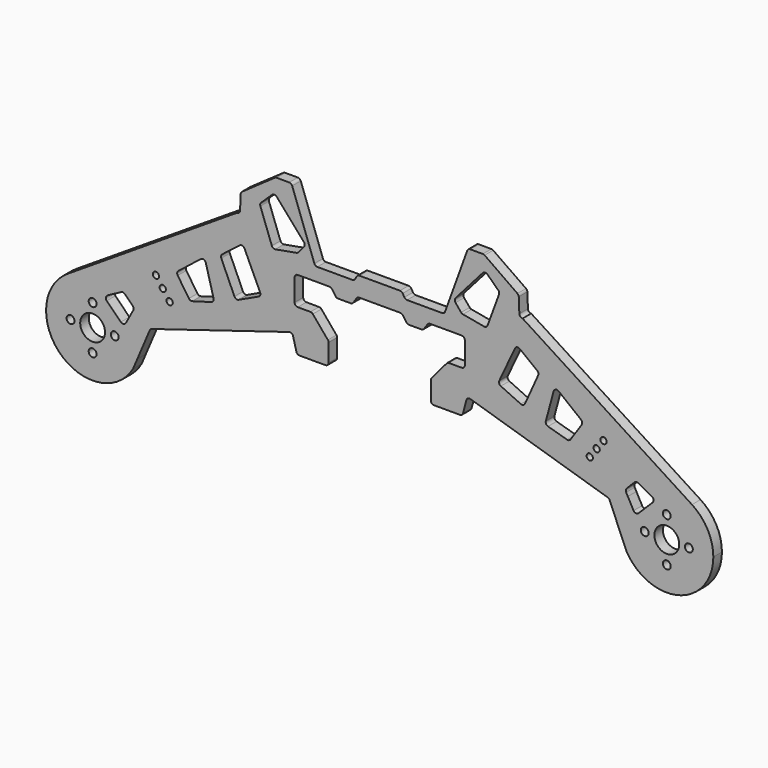
from build123d import *

# Parameters (mm, degrees)
F0_R     = 1
F0_R_2   = 1.25
F0_R_3   = 3.9333333333
F1_DEPTH = 3.4


# Not quite as in the source:
# - a feature names something its author has since deleted; it is built from what else it names


with BuildPart() as f1:
    # F0 (on Front) → F1 (new body)
    with BuildSketch(Plane.XZ):
        with BuildLine():
            Line((-8.2982365832, 14.9417242708), (-61.9791285384, 49.42693132))
            ThreePointArc((-61.9791285384, 49.42693132), (-62.6848131058, 49.6987576936), (-62.9984126547, 50.3868969303))
            Line((-62.9984126547, 50.3868969303), (-63.1852708125, 55.0742351752))
            ThreePointArc((-63.1852708125, 55.0742351752), (-63.3068405454, 55.5137289261), (-63.6109007347, 55.8535544083))
            Line((-63.6109007347, 55.8535544083), (-74.0052830565, 63.131779265))
            ThreePointArc((-74.0052830565, 63.131779265), (-74.2781536934, 63.2663441715), (-74.5788594929, 63.3126272207))
            Line((-74.5788594929, 63.3126272207), (-78.5633531658, 63.3126272207))
            ThreePointArc((-78.5633531658, 63.3126272207), (-79.1369296021, 63.131779265), (-79.5030457866, 62.6546473641))
            Line((-79.5030457866, 62.6546473641), (-86.5485187746, 43.2973694201))
            ThreePointArc((-86.5485187746, 43.2973694201), (-86.914634959, 42.8202375192), (-87.4882113954, 42.6393895635))
            Line((-87.4882113954, 42.6393895635), (-98.5779405442, 42.6393895635))
            ThreePointArc((-98.5779405442, 42.6393895635), (-99.0779405442, 42.7733641597), (-99.443965948, 43.1393895635))
            Line((-99.443965948, 43.1393895635), (-99.9635811902, 44.0393895635))
            ThreePointArc((-99.9635811902, 44.0393895635), (-100.329606594, 44.4054149672), (-100.829606594, 44.5393895635))
            Line((-100.829606594, 44.5393895635), (-107.2522563248, 44.5393895635))
            Line((-107.2522563248, 44.5393895635), (-113.6749060556, 44.5393895635))
            ThreePointArc((-113.6749060556, 44.5393895635), (-114.1749060556, 44.4054149672), (-114.5409314594, 44.0393895635))
            Line((-114.5409314594, 44.0393895635), (-115.0605467017, 43.1393895635))
            ThreePointArc((-115.0605467017, 43.1393895635), (-115.4265721055, 42.7733641597), (-115.9265721055, 42.6393895635))
            Line((-115.9265721055, 42.6393895635), (-127.0163012543, 42.6393895635))
            ThreePointArc((-127.0163012543, 42.6393895635), (-127.5898776906, 42.8202375192), (-127.9559938751, 43.2973694201))
            Line((-127.9559938751, 43.2973694201), (-135.0014668631, 62.6546473641))
            ThreePointArc((-135.0014668631, 62.6546473641), (-135.3675830475, 63.131779265), (-135.9411594839, 63.3126272207))
            Line((-135.9411594839, 63.3126272207), (-139.9256531568, 63.3126272207))
            ThreePointArc((-139.9256531568, 63.3126272207), (-140.2263589563, 63.2663441715), (-140.4992295931, 63.131779265))
            Line((-140.4992295931, 63.131779265), (-150.8936119149, 55.8535544083))
            ThreePointArc((-150.8936119149, 55.8535544083), (-151.1976721043, 55.5137289261), (-151.3192418372, 55.0742351752))
            Line((-151.3192418372, 55.0742351752), (-151.5060999949, 50.3868969303))
            ThreePointArc((-151.5060999949, 50.3868969303), (-151.8196995438, 49.6987576936), (-152.5253841113, 49.42693132))
            Line((-152.5253841113, 49.42693132), (-206.2062760664, 14.9417242708))
            ThreePointArc((-206.2062760664, 14.9417242708), (-198.1780596026, 17.281718999), (-190.1678289018, 14.8808776804))
            Line((-190.1678289018, 14.8808776804), (-189.1965146494, 15.4060313881))
            ThreePointArc((-189.1965146494, 15.4060313881), (-188.576544649, 15.5158937889), (-188.01380745, 15.2334767332))
            Line((-188.01380745, 15.2334767332), (-185.5323660974, 12.7520353807))
            ThreePointArc((-185.5323660974, 12.7520353807), (-185.2499490417, 12.1892981816), (-185.3598114425, 11.5693281812))
            Line((-185.3598114425, 11.5693281812), (-185.8849651503, 10.5980139288))
            ThreePointArc((-185.8849651503, 10.5980139288), (-184.0969913909, 6.7397922977), (-183.4840176852, 2.5318251454))
            ThreePointArc((-183.4840176852, 2.5318251454), (-183.6340282552, 0.4335380721), (-184.0810086875, -1.6220689687))
            Line((-184.0810086875, -1.6220689687), (-180.1264152738, 7.694369281))
            ThreePointArc((-180.1264152738, 7.694369281), (-179.8750410267, 8.0467829779), (-179.4982821251, 8.2599429084))
            Line((-179.4982821251, 8.2599429084), (-135.98817339, 21.5623181023))
            ThreePointArc((-135.98817339, 21.5623181023), (-135.2109920651, 21.4806330535), (-134.729875859, 20.8648323915))
            Line((-134.729875859, 20.8648323915), (-133.6435753937, 16.8107038626))
            ThreePointArc((-133.6435753937, 16.8107038626), (-133.2864109964, 16.2761695674), (-132.6776495674, 16.0695229077))
            Line((-132.6776495674, 16.0695229077), (-124.4449765554, 16.0695229077))
            ThreePointArc((-124.4449765554, 16.0695229077), (-123.7378697742, 16.3624161265), (-123.4449765554, 17.0695229077))
            Line((-123.4449765554, 17.0695229077), (-123.4449765554, 22.7055526735))
            ThreePointArc((-123.4449765554, 22.7055526735), (-123.5052839346, 23.0475728168), (-123.6789321123, 23.3483402831))
            Line((-123.6789321123, 23.3483402831), (-128.4482375504, 29.0321771731))
            ThreePointArc((-128.4482375504, 29.0321771731), (-128.7916637317, 29.2956973505), (-129.2142819935, 29.3893895635))
            Line((-129.2142819935, 29.3893895635), (-133.2142819935, 29.3893895635))
            ThreePointArc((-133.2142819935, 29.3893895635), (-133.9213887747, 29.6822827823), (-134.2142819935, 30.3893895635))
            Line((-134.2142819935, 30.3893895635), (-134.2142819935, 37.3893895635))
            ThreePointArc((-134.2142819935, 37.3893895635), (-133.9213887747, 38.0964963446), (-133.2142819935, 38.3893895635))
            Line((-133.2142819935, 38.3893895635), (-123.2142819935, 38.3893895635))
            ThreePointArc((-123.2142819935, 38.3893895635), (-122.7525333802, 38.2764003966), (-122.3951299492, 37.9629659998))
            Line((-122.3951299492, 37.9629659998), (-121.2715706276, 36.3583569942))
            ThreePointArc((-121.2715706276, 36.3583569942), (-120.9141671966, 36.0449225974), (-120.4524185833, 35.9319334306))
            Line((-120.4524185833, 35.9319334306), (-116.4935526844, 35.9319334306))
            ThreePointArc((-116.4935526844, 35.9319334306), (-116.0318040712, 36.0449225974), (-115.6744006401, 36.3583569942))
            Line((-115.6744006401, 36.3583569942), (-114.5508413186, 37.9629659998))
            ThreePointArc((-114.5508413186, 37.9629659998), (-114.1934378875, 38.2764003966), (-113.7316892743, 38.3893895635))
            Line((-113.7316892743, 38.3893895635), (-107.2522563248, 38.3893895635))
            Line((-107.2522563248, 38.3893895635), (-100.7728233754, 38.3893895635))
            ThreePointArc((-100.7728233754, 38.3893895635), (-100.3110747621, 38.2764003966), (-99.9536713311, 37.9629659998))
            Line((-99.9536713311, 37.9629659998), (-98.8301120095, 36.3583569942))
            ThreePointArc((-98.8301120095, 36.3583569942), (-98.4727085785, 36.0449225974), (-98.0109599652, 35.9319334306))
            Line((-98.0109599652, 35.9319334306), (-94.0520940663, 35.9319334306))
            ThreePointArc((-94.0520940663, 35.9319334306), (-93.5903454531, 36.0449225974), (-93.232942022, 36.3583569942))
            Line((-93.232942022, 36.3583569942), (-92.1093827005, 37.9629659998))
            ThreePointArc((-92.1093827005, 37.9629659998), (-91.7519792694, 38.2764003966), (-91.2902306562, 38.3893895635))
            Line((-91.2902306562, 38.3893895635), (-81.2902306562, 38.3893895635))
            ThreePointArc((-81.2902306562, 38.3893895635), (-80.583123875, 38.0964963446), (-80.2902306562, 37.3893895635))
            Line((-80.2902306562, 37.3893895635), (-80.2902306562, 30.3893895635))
            ThreePointArc((-80.2902306562, 30.3893895635), (-80.583123875, 29.6822827823), (-81.2902306562, 29.3893895635))
            Line((-81.2902306562, 29.3893895635), (-85.2902306562, 29.3893895635))
            ThreePointArc((-85.2902306562, 29.3893895635), (-85.7128489179, 29.2956973505), (-86.0562750993, 29.0321771731))
            Line((-86.0562750993, 29.0321771731), (-90.8255805374, 23.3483402831))
            ThreePointArc((-90.8255805374, 23.3483402831), (-90.999228715, 23.0475728168), (-91.0595360942, 22.7055526735))
            Line((-91.0595360942, 22.7055526735), (-91.0595360942, 17.0695229077))
            ThreePointArc((-91.0595360942, 17.0695229077), (-90.7666428754, 16.3624161265), (-90.0595360942, 16.0695229077))
            Line((-90.0595360942, 16.0695229077), (-81.8268630822, 16.0695229077))
            ThreePointArc((-81.8268630822, 16.0695229077), (-81.2181016532, 16.2761695674), (-80.8609372559, 16.8107038626))
            Line((-80.8609372559, 16.8107038626), (-79.7746367906, 20.8648323915))
            ThreePointArc((-79.7746367906, 20.8648323915), (-79.2935205846, 21.4806330535), (-78.5163392596, 21.5623181023))
            Line((-78.5163392596, 21.5623181023), (-35.0062305246, 8.2599429084))
            ThreePointArc((-35.0062305246, 8.2599429084), (-34.629471623, 8.0467829779), (-34.3780973759, 7.694369281))
            Line((-34.3780973759, 7.694369281), (-30.4235039621, -1.6220689687))
            ThreePointArc((-30.4235039621, -1.6220689687), (-30.8623564932, 4.6859089703), (-28.6195474994, 10.5980139288))
            Line((-28.6195474994, 10.5980139288), (-29.1447012071, 11.5693281812))
            ThreePointArc((-29.1447012071, 11.5693281812), (-29.2545636079, 12.1892981816), (-28.9721465522, 12.7520353807))
            Line((-28.9721465522, 12.7520353807), (-26.4907051997, 15.2334767332))
            ThreePointArc((-26.4907051997, 15.2334767332), (-25.9279680006, 15.5158937889), (-25.3079980002, 15.4060313881))
            Line((-25.3079980002, 15.4060313881), (-24.3366837478, 14.8808776804))
            ThreePointArc((-24.3366837478, 14.8808776804), (-16.326453047, 17.281718999), (-8.2982365832, 14.9417242708))
        make_face()
        with Locations((-173.8244922322, 17.708704086)):
            Circle(F0_R, mode=Mode.SUBTRACT)
        with Locations((-176.002322044, 20.6961818324)):
            Circle(F0_R, mode=Mode.SUBTRACT)
        with Locations((-178.1801518558, 23.6836595789)):
            Circle(F0_R, mode=Mode.SUBTRACT)
        with Locations((-40.6800204174, 17.708704086)):
            Circle(F0_R, mode=Mode.SUBTRACT)
        with Locations((-38.5021906056, 20.6961818324)):
            Circle(F0_R, mode=Mode.SUBTRACT)
        with Locations((-36.3243607939, 23.6836595789)):
            Circle(F0_R, mode=Mode.SUBTRACT)
        with BuildLine():
            Line((-160.5823523456, 21.9218021251), (-166.625047012, 20.1887688389))
            ThreePointArc((-166.625047012, 20.1887688389), (-167.243951709, 20.2107622631), (-167.7312221572, 20.5929850319))
            Line((-167.7312221572, 20.5929850319), (-171.2672607403, 25.8649401874))
            ThreePointArc((-171.2672607403, 25.8649401874), (-171.4248117311, 26.5761574447), (-171.0580559772, 27.205555982))
            Line((-171.0580559772, 27.205555982), (-163.960280146, 32.8332256047))
            ThreePointArc((-163.960280146, 32.8332256047), (-163.0262819721, 32.9994898925), (-162.3737234369, 32.3108943943))
            Line((-162.3737234369, 32.3108943943), (-159.8927660185, 23.1443029023))
            ThreePointArc((-159.8927660185, 23.1443029023), (-159.987049053, 22.3917451518), (-160.5823523456, 21.9218021251))
        make_face(mode=Mode.SUBTRACT)
        with BuildLine():
            Line((-157.1668727058, 36.3584228689), (-151.6300301262, 40.6507917671))
            ThreePointArc((-151.6300301262, 40.6507917671), (-150.7820649144, 40.8323962189), (-150.1110333324, 40.2830859301))
            Line((-150.1110333324, 40.2830859301), (-145.1462509097, 29.6360756657))
            ThreePointArc((-145.1462509097, 29.6360756657), (-145.1128660759, 28.8714372607), (-145.629940435, 28.307149617))
            Line((-145.629940435, 28.307149617), (-151.9604140529, 25.3552012892))
            ThreePointArc((-151.9604140529, 25.3552012892), (-152.7320819557, 25.3244048408), (-153.2955697507, 25.8525158881))
            Line((-153.2955697507, 25.8525158881), (-157.4667211351, 35.1591055821))
            ThreePointArc((-157.4667211351, 35.1591055821), (-157.5243225624, 35.8106489423), (-157.1668727058, 36.3584228689))
        make_face(mode=Mode.SUBTRACT)
        with BuildLine():
            Line((-131.2632317355, 46.9035901921), (-133.0417308846, 44.7654929954))
            ThreePointArc((-133.0417308846, 44.7654929954), (-133.3068150219, 44.541115727), (-133.6326541752, 44.4209341783))
            Line((-133.6326541752, 44.4209341783), (-140.3211977924, 43.211949673))
            ThreePointArc((-140.3211977924, 43.211949673), (-140.9953494339, 43.3278404753), (-141.4372863809, 43.8499543026))
            Line((-141.4372863809, 43.8499543026), (-145.0733456256, 53.7081270257))
            ThreePointArc((-145.0733456256, 53.7081270257), (-145.1098099647, 54.2777769012), (-144.8286934499, 54.7745707555))
            Line((-144.8286934499, 54.7745707555), (-141.3709317505, 58.1035511138))
            ThreePointArc((-141.3709317505, 58.1035511138), (-140.6356224072, 58.3822846563), (-139.9261270555, 58.0431850192))
            Line((-139.9261270555, 58.0431850192), (-131.2807867439, 48.2031136398))
            ThreePointArc((-131.2807867439, 48.2031136398), (-131.0321183971, 47.5565925544), (-131.2632317355, 46.9035901921))
        make_face(mode=Mode.SUBTRACT)
        with BuildLine():
            ThreePointArc((-61.208942899, 25.8525158881), (-61.7724306939, 25.3244048408), (-62.5440985967, 25.3552012892))
            Line((-62.5440985967, 25.3552012892), (-68.8745722147, 28.307149617))
            ThreePointArc((-68.8745722147, 28.307149617), (-69.3916465737, 28.8714372607), (-69.35826174, 29.6360756657))
            Line((-69.35826174, 29.6360756657), (-64.3934793172, 40.2830859301))
            ThreePointArc((-64.3934793172, 40.2830859301), (-63.7224477352, 40.8323962189), (-62.8744825234, 40.6507917671))
            Line((-62.8744825234, 40.6507917671), (-57.3376399438, 36.3584228689))
            ThreePointArc((-57.3376399438, 36.3584228689), (-56.9801900873, 35.8106489423), (-57.0377915146, 35.1591055821))
            Line((-57.0377915146, 35.1591055821), (-61.208942899, 25.8525158881))
        make_face(mode=Mode.SUBTRACT)
        with BuildLine():
            Line((-43.2372519093, 25.8649401874), (-46.7732904924, 20.5929850319))
            ThreePointArc((-46.7732904924, 20.5929850319), (-47.2605609406, 20.2107622631), (-47.8794656376, 20.1887688389))
            Line((-47.8794656376, 20.1887688389), (-53.9221603041, 21.9218021251))
            ThreePointArc((-53.9221603041, 21.9218021251), (-54.5174635967, 22.3917451518), (-54.6117466311, 23.1443029023))
            Line((-54.6117466311, 23.1443029023), (-52.1307892128, 32.3108943943))
            ThreePointArc((-52.1307892128, 32.3108943943), (-51.4782306775, 32.9994898925), (-50.5442325037, 32.8332256047))
            Line((-50.5442325037, 32.8332256047), (-43.4464566724, 27.205555982))
            ThreePointArc((-43.4464566724, 27.205555982), (-43.0797009186, 26.5761574447), (-43.2372519093, 25.8649401874))
        make_face(mode=Mode.SUBTRACT)
        with BuildLine():
            Line((-83.2237259058, 48.2031136398), (-74.5783855942, 58.0431850192))
            ThreePointArc((-74.5783855942, 58.0431850192), (-73.8688902424, 58.3822846563), (-73.1335808991, 58.1035511138))
            Line((-73.1335808991, 58.1035511138), (-69.6758191998, 54.7745707555))
            ThreePointArc((-69.6758191998, 54.7745707555), (-69.394702685, 54.2777769012), (-69.4311670241, 53.7081270257))
            Line((-69.4311670241, 53.7081270257), (-73.0672262687, 43.8499543026))
            ThreePointArc((-73.0672262687, 43.8499543026), (-73.5091632157, 43.3278404753), (-74.1833148572, 43.211949673))
            Line((-74.1833148572, 43.211949673), (-80.8718584745, 44.4209341783))
            ThreePointArc((-80.8718584745, 44.4209341783), (-81.1976976277, 44.541115727), (-81.462781765, 44.7654929954))
            Line((-81.462781765, 44.7654929954), (-83.2412809141, 46.9035901921))
            ThreePointArc((-83.2412809141, 46.9035901921), (-83.4723942526, 47.5565925544), (-83.2237259058, 48.2031136398))
        make_face(mode=Mode.SUBTRACT)
        with BuildLine():
            ThreePointArc((-1.5204949644, 2.5318251454), (-3.3253547349, 9.6018919371), (-8.2982365832, 14.9417242708))
            ThreePointArc((-8.2982365832, 14.9417242708), (-16.326453047, 17.281718999), (-24.3366837478, 14.8808776804))
            Line((-24.3366837478, 14.8808776804), (-20.9862185313, 13.0694050013))
            ThreePointArc((-20.9862185313, 13.0694050013), (-20.4722951127, 12.3341131473), (-20.7547121684, 11.482636784))
            Line((-20.7547121684, 11.482636784), (-25.221306603, 7.0160423494))
            ThreePointArc((-25.221306603, 7.0160423494), (-26.0727829663, 6.7336252937), (-26.8080748203, 7.2475487123))
            Line((-26.8080748203, 7.2475487123), (-28.6195474994, 10.5980139288))
            ThreePointArc((-28.6195474994, 10.5980139288), (-30.8623564932, 4.6859089703), (-30.4235039621, -1.6220689687))
            Line((-30.4235039621, -1.6220689687), (-29.0900624945, -4.7634602048))
            ThreePointArc((-29.0900624945, -4.7634602048), (-12.4973080534, -11.7274020614), (-1.5204949644, 2.5318251454))
        make_face()
        with Locations((-16.2704949644, -4.4681748546)):
            Circle(F0_R_2, mode=Mode.SUBTRACT)
        with Locations((-23.2704949644, 2.5318251454)):
            Circle(F0_R_2, mode=Mode.SUBTRACT)
        with Locations((-16.2704949644, 2.5318251454)):
            Circle(F0_R_3, mode=Mode.SUBTRACT)
        with Locations((-9.2704949644, 2.5318251454)):
            Circle(F0_R_2, mode=Mode.SUBTRACT)
        with Locations((-16.2704949644, 9.5318251454)):
            Circle(F0_R_2, mode=Mode.SUBTRACT)
        with BuildLine():
            ThreePointArc((-190.1678289018, 14.8808776804), (-198.1780596026, 17.281718999), (-206.2062760664, 14.9417242708))
            ThreePointArc((-206.2062760664, 14.9417242708), (-208.38033107, -8.1740061954), (-185.4144501551, -4.7634602048))
            Line((-185.4144501551, -4.7634602048), (-184.0810086875, -1.6220689687))
            ThreePointArc((-184.0810086875, -1.6220689687), (-183.6340282552, 0.4335380721), (-183.4840176852, 2.5318251454))
            ThreePointArc((-183.4840176852, 2.5318251454), (-184.0969913909, 6.7397922977), (-185.8849651503, 10.5980139288))
            Line((-185.8849651503, 10.5980139288), (-187.6964378294, 7.2475487123))
            ThreePointArc((-187.6964378294, 7.2475487123), (-188.4317296833, 6.7336252937), (-189.2832060467, 7.0160423494))
            Line((-189.2832060467, 7.0160423494), (-193.7498004812, 11.482636784))
            ThreePointArc((-193.7498004812, 11.482636784), (-194.0322175369, 12.3341131473), (-193.5182941183, 13.0694050013))
            Line((-193.5182941183, 13.0694050013), (-190.1678289018, 14.8808776804))
        make_face()
        with Locations((-198.2340176852, -4.4681748546)):
            Circle(F0_R_2, mode=Mode.SUBTRACT)
        with Locations((-205.2340176852, 2.5318251454)):
            Circle(F0_R_2, mode=Mode.SUBTRACT)
        with Locations((-198.2340176852, 2.5318251454)):
            Circle(F0_R_3, mode=Mode.SUBTRACT)
        with Locations((-191.2340176852, 2.5318251454)):
            Circle(F0_R_2, mode=Mode.SUBTRACT)
        with Locations((-198.2340176852, 9.5318251454)):
            Circle(F0_R_2, mode=Mode.SUBTRACT)
    extrude(amount=F1_DEPTH)


solid = f1.part
